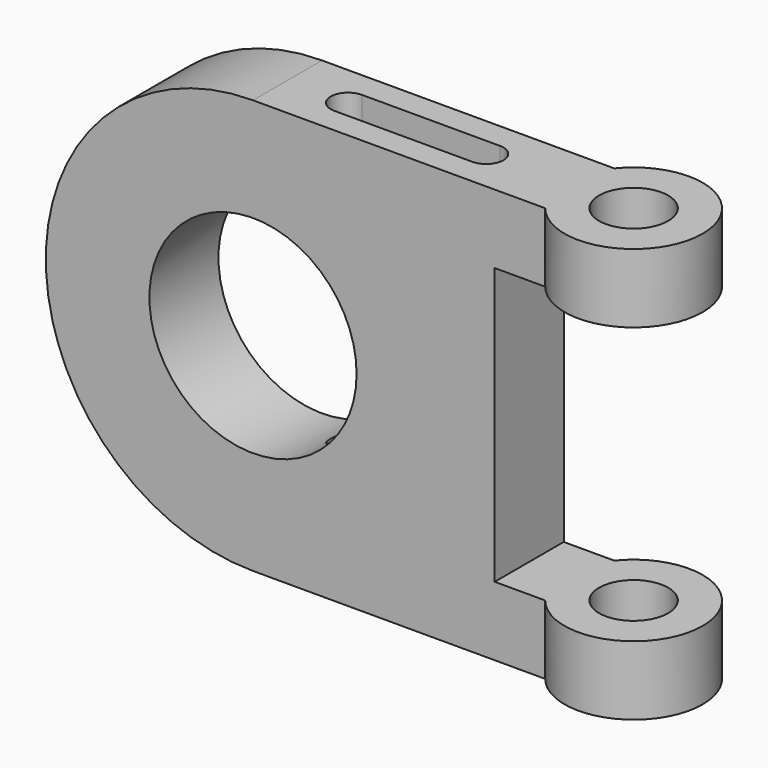
from build123d import *

# Parameters (mm, degrees)
F0_R     = 38.1
F1_DEPTH = 15.875
F3_DEPTH = 152.4
F4_R     = 12.7
F5_DEPTH = 25.4


# Not quite as in the source:
# - a feature names something its author has since deleted; it is built from what else it names


with BuildPart() as f1:
    # F0 (on Front) → F1 (new body, symmetric)
    with BuildSketch(Plane.XZ):
        with BuildLine():
            Line((70.8614879427, 70.3741200164), (-36.6122665732, 70.3741200164))
            ThreePointArc((-36.6122665732, 70.3741200164), (-112.8122614121, -5.8258799836), (-36.6122665732, -82.0258799836))
            Line((-36.6122665732, -82.0258799836), (70.8614879427, -82.0258799836))
            Line((70.8614879427, -82.0258799836), (70.8614879427, -56.6258799836))
            Line((70.8614879427, -56.6258799836), (52.2877385879, -56.6258799836))
            Line((52.2877385879, -56.6258799836), (52.2877385879, 44.9741200164))
            Line((52.2877385879, 44.9741200164), (70.8614879427, 44.9741200164))
            Line((70.8614879427, 44.9741200164), (70.8614879427, 70.3741200164))
        make_face()
        with Locations((-36.6122614121, -5.8258799836)):
            Circle(F0_R, mode=Mode.SUBTRACT)
    extrude(amount=F1_DEPTH, both=True)

    # F2 (on face) → F3 (cut)
    with BuildSketch(Plane.XY.offset(70.3741200164)):
        with BuildLine():
            Line((36.4952879427, 6.2992834322), (-14.3047120573, 6.2992834322))
            ThreePointArc((-14.3047120573, 6.2992834322), (-20.6547120573, -0.0507165678), (-14.3047120573, -6.4007165678))
            Line((-14.3047120573, -6.4007165678), (36.4952879427, -6.4007165678))
            ThreePointArc((36.4952879427, -6.4007165678), (42.8452879427, -0.0507165678), (36.4952879427, 6.2992834322))
        make_face()
    extrude(amount=-F3_DEPTH, mode=Mode.SUBTRACT)

    # F4 (on face) → F5 (join)
    with BuildSketch(Plane.XY.offset(70.3741200164)):
        with BuildLine():
            Line((70.8614879427, 15.875), (70.8614879427, -15.875))
            ThreePointArc((70.8614879427, -15.875), (116.0893565876, 0), (70.8614879427, 15.875))
        make_face()
        with Locations((90.6893565876, 0)):
            Circle(F4_R, mode=Mode.SUBTRACT)
    extrude(amount=-F5_DEPTH)

    # F7: F1 across plane


with BuildPart() as f1_1:
    add(f1.part)
    add(f1.part.mirror(Plane(origin=(52.2877385879, -15.875, -5.8258799836), x_dir=(1, 0, 0), z_dir=(0, 0, -1))))


solid = f1_1.part
